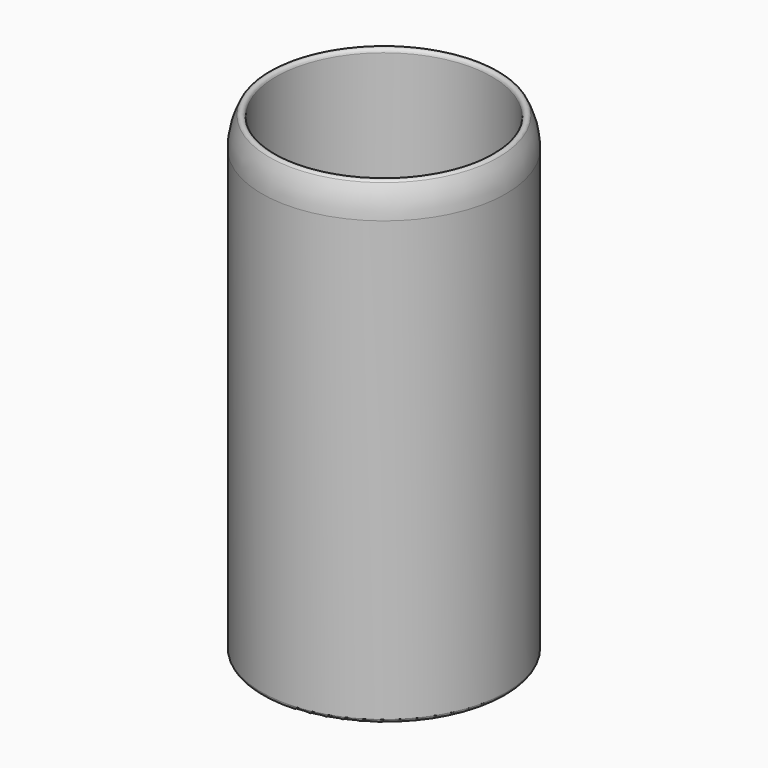
from build123d import *

# Parameters (mm, degrees)
F0_R     = 436.7191768954
F1_DEPTH = 1727.2
F2_T     = -50
F4_R     = 12.7


# Not quite as in the source:
# - a fillet or chamfer that OpenCascade refuses, or shapes differently, is made with other operations: its cross-section is extruded or revolved along the edge and cut away or added


with BuildPart() as f1:
    # F0 (on Top) → F1 (new body)
    with BuildSketch(Plane.XY):
        Circle(F0_R)
    extrude(amount=F1_DEPTH)

    # F2
    f2_openings = [f1.faces().sort_by_distance(p)[0] for p in [
        (0, 0, 1727.2),
    ]]
    offset(amount=F2_T, openings=f2_openings)

    # F3: fillet of radius 233.0198930403 on 1 edges, made by hand

    # F3_s1 → F3_t2 (revolve, cut)
    with BuildSketch(Plane.XZ):
        with BuildLine():
            ThreePointArc((436.7191768954, 1582.9710524755), (423.8646154278, 1659.2959981093), (386.7191768954, 1727.2))
            Line((386.7191768954, 1727.2), (436.7191768954, 1727.2))
            Line((436.7191768954, 1727.2), (436.7191768954, 1582.9710524755))
        make_face()
    revolve(axis=Axis((0, 0, 1727.2), (0, 0, 1)), mode=Mode.SUBTRACT)

    # F4
    f4_edges = [f1.edges().sort_by_distance(p)[0] for p in [
        (-436.719177, 0, 0),
        (-386.719177, 0, 50),
        (386.719177, 0, 888.6),
        (-386.719177, 0, 1727.2),
    ]]
    fillet(f4_edges, radius=F4_R)


solid = f1.part
